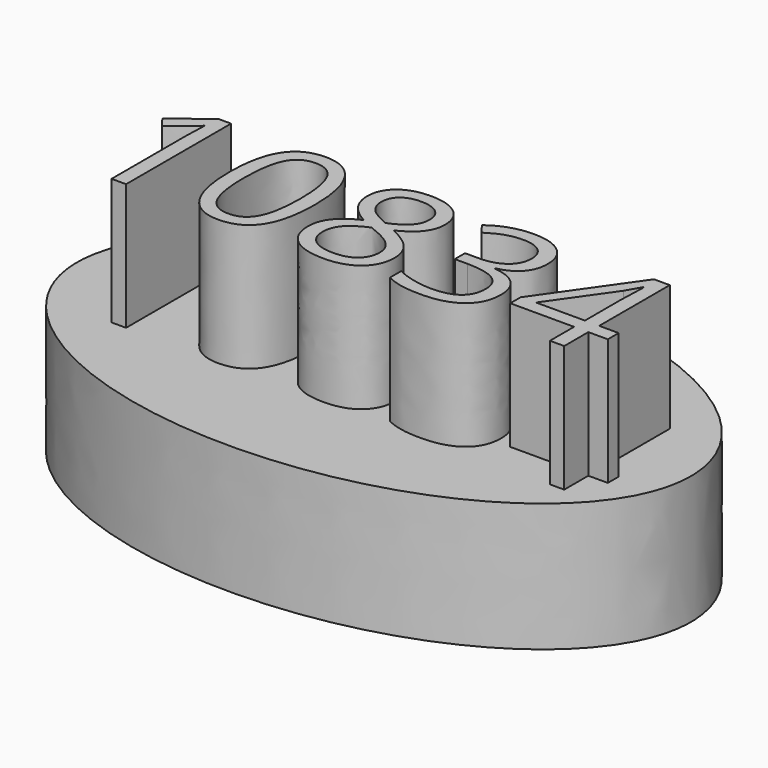
from build123d import *

# Parameters (mm, degrees)
F1_DEPTH     = 33.02
F2_TEXT_SIZE = 47.2632249663
F3_DEPTH     = 32.512


# Not quite as in the source:
# - Text() gives the source's letters only with a copy of the font that has no kerning and outlines rounded to 1/6400 em; it was checked with that copy


with BuildPart() as f1:
    # F0 (on Top) → F1 (new body)
    with BuildSketch(Plane.XY):
        with BuildLine():
            add(Edge.make_bspline(
                [(77.1564915776, 3.3871850464), (73.7140641033, 81.8020406828), (-40.299459526, 37.513835295), (-154.3129831553, -6.7743700929), (-36.8570320516, -40.9010203414), (80.598919052, -75.0276705899), (77.1564915776, 3.3871850464)],
                knots=[0, 0, 0, 2.0943951024, 2.0943951024, 4.1887902048, 4.1887902048, 6.2831853072, 6.2831853072, 6.2831853072], degree=2, weights=[1, 0.5, 1, 0.5, 1, 0.5, 1]))
        make_face()
    extrude(amount=-F1_DEPTH)

    # F2 (on face) → F3 (join)
    with BuildSketch(Plane.XY):
        with Locations((-68.1869691139, -18.2869281896)):
            Text('10834', F2_TEXT_SIZE, font='Open Sans', text_align=(TextAlign.LEFT, TextAlign.BOTTOM))
    extrude(amount=F3_DEPTH)


solid = f1.part
